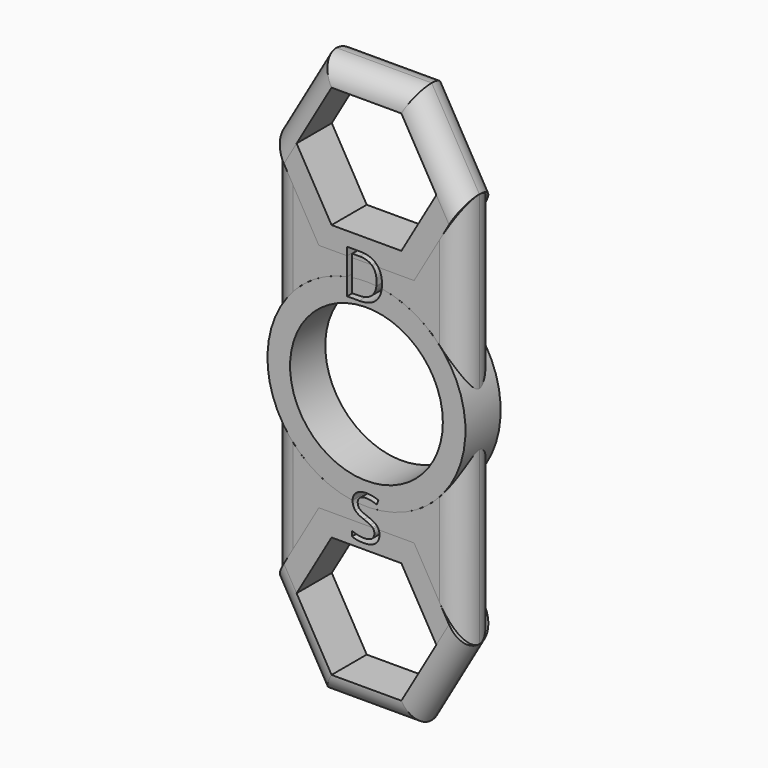
from build123d import *

# Parameters (mm, degrees)
F2_DEPTH = 6.35
F0_R     = 14.2875
F0_R_2   = 11.0236
F3_R     = 3.17499
F3_2_R   = 3.17499
F3_3_R   = 3.17499
F3_4_R   = 3.17499
F6_DEPTH = 25.4
F7_DEPTH = 25.4


# Not quite as in the source:
# - a fillet or chamfer is up to 0.001 mm smaller than in the source, because OpenCascade refuses the exact size


with BuildPart() as f2:
    # F1 (on Front) → F2 (new body)
    with BuildSketch(Plane.XZ):
        with BuildLine():
            Line((13.7481532851, -28.575), (13.7481532851, -3.8885649667))
            ThreePointArc((13.7481532851, -3.8885649667), (0, -14.2875), (-13.7481532851, -3.8885649667))
            Line((-13.7481532851, -3.8885649667), (-13.7481532851, -28.575))
            Line((-13.7481532851, -28.575), (-10.3111149312, -22.6218749436))
            Line((-10.3111149312, -22.6218749436), (-6.8740766425, -16.66875))
            Line((-6.8740766425, -16.66875), (0, -16.66875))
            Line((0, -16.66875), (6.8740766425, -16.66875))
            Line((6.8740766425, -16.66875), (10.3111148375, -22.6218747812))
            Line((10.3111148375, -22.6218747812), (13.7481532851, -28.575))
        make_face()
    extrude(amount=F2_DEPTH)

    # F3#3 (radius 3.175 in the source; OpenCascade refuses exactly that, so slightly less here)
    f3_3_edges = [f2.edges().sort_by_distance(p)[0] for p in [
        (13.748153, -6.35, -16.231782),
        (-13.748153, -6.35, -16.231782),
        (13.748153, 0, -16.231782),
        (-13.748153, 0, -16.231782),
    ]]
    fillet(f3_3_edges, radius=F3_3_R)


with BuildPart() as f2b:
    # F1 (on Front) → F2, piece 2 (new body)
    with BuildSketch(Plane.XZ):
        with BuildLine():
            Line((13.7481532851, 3.8885649667), (13.7481532851, 28.575))
            Line((13.7481532851, 28.575), (10.3111149612, 22.6218749955))
            Line((10.3111149612, 22.6218749955), (6.8740766425, 16.66875))
            Line((6.8740766425, 16.66875), (0, 16.66875))
            Line((0, 16.66875), (-6.8740766425, 16.66875))
            Line((-6.8740766425, 16.66875), (-10.3111150377, 22.6218751279))
            Line((-10.3111150377, 22.6218751279), (-13.7481532851, 28.575))
            Line((-13.7481532851, 28.575), (-13.7481532851, 3.8885649667))
            ThreePointArc((-13.7481532851, 3.8885649667), (0, 14.2875), (13.7481532851, 3.8885649667))
        make_face()
    extrude(amount=F2_DEPTH)

    # F3#2 (radius 3.175 in the source; OpenCascade refuses exactly that, so slightly less here)
    f3_2_edges = [f2b.edges().sort_by_distance(p)[0] for p in [
        (13.748153, -6.35, 16.231782),
        (-13.748153, -6.35, 16.231782),
        (13.748153, 0, 16.231782),
        (-13.748153, 0, 16.231782),
    ]]
    fillet(f3_2_edges, radius=F3_2_R)


with BuildPart() as f2c:
    # F0 (on Front) → F2, piece 3 (new body)
    with BuildSketch(Plane.XZ):
        Circle(F0_R)
        Circle(F0_R_2, mode=Mode.SUBTRACT)
    extrude(amount=F2_DEPTH)


with BuildPart() as f2d:
    # F0 (on Front) → F2, piece 4 (new body)
    with BuildSketch(Plane.XZ):
        Polygon((6.8740766425, -16.66875), (-6.8740766425, -16.66875), (-13.7481532851, -28.575), (-6.8740766425, -40.48125), (6.8740766425, -40.48125), (13.7481532851, -28.575), align=None)
        Polygon((-10.0819790757, -28.575), (-5.0409895379, -19.84375), (5.0409895379, -19.84375), (10.0819790757, -28.575), (5.0409895379, -37.30625), (-5.0409895379, -37.30625), align=None, mode=Mode.SUBTRACT)
    extrude(amount=F2_DEPTH)

    # F3#4 (radius 3.175 in the source; OpenCascade refuses exactly that, so slightly less here)
    f3_4_edges = [f2d.edges().sort_by_distance(p)[0] for p in [
        (10.311115, -6.35, -34.528125),
        (0, -6.35, -40.48125),
        (-10.311115, -6.35, -34.528125),
        (10.311115, 0, -34.528125),
        (0, 0, -40.48125),
        (-10.311115, 0, -34.528125),
    ]]
    fillet(f3_4_edges, radius=F3_4_R)


with BuildPart() as f2e:
    # F0 (on Front) → F2, piece 5 (new body)
    with BuildSketch(Plane.XZ):
        Polygon((-6.8740766425, 40.48125), (-13.7481532851, 28.575), (-6.8740766425, 16.66875), (6.8740766425, 16.66875), (13.7481532851, 28.575), (6.8740766425, 40.48125), align=None)
        Polygon((-10.0819790757, 28.575), (-5.0409895379, 37.30625), (5.0409895379, 37.30625), (10.0819790757, 28.575), (5.0409895379, 19.84375), (-5.0409895379, 19.84375), align=None, mode=Mode.SUBTRACT)
    extrude(amount=F2_DEPTH)

    # F3 (radius 3.175 in the source; OpenCascade refuses exactly that, so slightly less here)
    f3_edges = [f2e.edges().sort_by_distance(p)[0] for p in [
        (-10.311115, -6.35, 34.528125),
        (0, -6.35, 40.48125),
        (10.311115, -6.35, 34.528125),
        (0, 0, 40.48125),
        (10.311115, 0, 34.528125),
        (-10.311115, 0, 34.528125),
    ]]
    fillet(f3_edges, radius=F3_R)


with BuildPart() as f6_tool:
    # F4 (on face) → F6 (new body)
    with BuildSketch(Plane.XZ.offset(6.35)):
        with BuildLine():
            Line((0.7356463616, 16.66875), (1.7117723609, 16.66875))
            add(Edge.make_bspline(
                [(1.4261315737, 17.0095994575), (1.5843296653, 16.8514013659), (1.7117723609, 16.66875)],
                knots=[0, 0, 0, 0.1944106639, 0.1944106639, 0.1944106639], degree=2))
            add(Edge.make_bspline(
                [(-0.8565886954, 17.8233310113), (0.6124000198, 17.8233310113), (1.4261315737, 17.0095994575)],
                knots=[0, 0, 0, 1, 1, 1], degree=2))
            Line((-0.8565886954, 17.8233310113), (-2.7858421677, 17.8233310113))
            Line((-2.7858421677, 17.8233310113), (-2.7858421677, 16.66875))
            Line((-2.7858421677, 16.66875), (-2.0541038864, 16.66875))
            Line((-2.0541038864, 16.66875), (-2.0541038864, 17.1894334419))
            Line((-2.0541038864, 17.1894334419), (-0.9902584003, 17.1894334419))
            add(Edge.make_bspline(
                [(0.7356463616, 16.66875), (0.1235530561, 17.1894334419), (-0.9902584003, 17.1894334419)],
                knots=[0.0867132539, 0.0867132539, 0.0867132539, 1, 1, 1], degree=2))
        make_face()
        with BuildLine():
            ThreePointArc((-2.7858421677, 14.0132701275), (-2.4207903425, 14.0809243435), (-2.0541038864, 14.13907046))
            Line((-2.0541038864, 14.13907046), (-2.0541038864, 16.66875))
            Line((-2.0541038864, 16.66875), (-2.7858421677, 16.66875))
            Line((-2.7858421677, 16.66875), (-2.7858421677, 14.0132701275))
        make_face()
        with BuildLine():
            add(Edge.make_bspline(
                [(2.2030186501, 14.1166343396), (2.0632995934, 13.0044799084), (1.3937476761, 12.3518303603)],
                knots=[0.2086754636, 0.2086754636, 0.2086754636, 1, 1, 1], degree=2))
            ThreePointArc((2.2030186501, 14.1166343396), (1.8208483174, 14.1709974121), (1.4373488308, 14.2150161656))
            add(Edge.make_bspline(
                [(0.8060143862, 12.8038268881), (1.329389377, 13.31517027), (1.4373488308, 14.2150161656)],
                knots=[0, 0, 0, 0.7937244697, 0.7937244697, 0.7937244697], degree=2))
            add(Edge.make_bspline(
                [(-1.1625131746, 12.1595940322), (0.1466231101, 12.1595940322), (0.8060143862, 12.8038268881)],
                knots=[0, 0, 0, 1, 1, 1], degree=2))
            Line((-1.1625131746, 12.1595940322), (-2.0541038864, 12.1595940322))
            Line((-2.0541038864, 12.1595940322), (-2.0541038864, 14.13907046))
            ThreePointArc((-2.0541038864, 14.13907046), (-2.4207903425, 14.0809243435), (-2.7858421677, 14.0132701275))
            Line((-2.7858421677, 14.0132701275), (-2.7858421677, 11.5270745009))
            Line((-2.7858421677, 11.5270745009), (-1.0412458135, 11.5270745009))
            add(Edge.make_bspline(
                [(1.3937476761, 12.3518303603), (0.5476322247, 11.5270745009), (-1.0412458135, 11.5270745009)],
                knots=[0, 0, 0, 1, 1, 1], degree=2))
        make_face()
        with BuildLine():
            add(Edge.make_bspline(
                [(2.2398631275, 14.7351474176), (2.2398631275, 14.4099139371), (2.2030186501, 14.1166343396)],
                knots=[0, 0, 0, 0.2086754636, 0.2086754636, 0.2086754636], degree=2))
            add(Edge.make_bspline(
                [(1.7117723609, 16.66875), (2.2398631275, 15.9118882642), (2.2398631275, 14.7351474176)],
                knots=[0.1944106639, 0.1944106639, 0.1944106639, 1, 1, 1], degree=2))
            Line((1.7117723609, 16.66875), (0.7356463616, 16.66875))
            add(Edge.make_bspline(
                [(0.847355532, 16.5651821398), (0.7937623941, 16.6193130015), (0.7356463616, 16.66875)],
                knots=[0, 0, 0, 0.0867132539, 0.0867132539, 0.0867132539], degree=2))
            add(Edge.make_bspline(
                [(1.4654056622, 14.7089646919), (1.4654056622, 15.9409308377), (0.847355532, 16.5651821398)],
                knots=[0, 0, 0, 1, 1, 1], degree=2))
            add(Edge.make_bspline(
                [(1.4373488308, 14.2150161656), (1.4654056622, 14.448870855), (1.4654056622, 14.7089646919)],
                knots=[0.7937244697, 0.7937244697, 0.7937244697, 1, 1, 1], degree=2))
            ThreePointArc((1.4373488308, 14.2150161656), (1.8208483174, 14.1709974121), (2.2030186501, 14.1166343396))
        make_face()
    extrude(amount=-F6_DEPTH)


with BuildPart() as f2b_1:
    add(f2b.part)

    # F6: cut by f6_tool
    add(f6_tool.part, mode=Mode.SUBTRACT)


with BuildPart() as f2c_1:
    add(f2c.part)

    # F6: cut by f6_tool
    add(f6_tool.part, mode=Mode.SUBTRACT)


with BuildPart() as f2e_1:
    add(f2e.part)

    # F6: cut by f6_tool
    add(f6_tool.part, mode=Mode.SUBTRACT)


with BuildPart() as f7_tool:
    # F5 (on face) → F7 (new body)
    with BuildSketch(Plane.XZ.offset(6.35)):
        with BuildLine():
            ThreePointArc((-2.0011550915, -14.1466616044), (-1.6310895837, -14.1940904259), (-1.2599118366, -14.2318403031))
            add(Edge.make_bspline(
                [(-1.2611806878, -14.1660674247), (-1.2611806878, -14.1995701631), (-1.2599118366, -14.2318403031)],
                knots=[0, 0, 0, 0.1025818921, 0.1025818921, 0.1025818921], degree=2))
            add(Edge.make_bspline(
                [(-0.9338966167, -13.4729142129), (-1.2611806878, -13.7223391261), (-1.2611806878, -14.1660674247)],
                knots=[0, 0, 0, 1, 1, 1], degree=2))
            add(Edge.make_bspline(
                [(-0.0250804274, -13.2234892997), (-0.6066125455, -13.2234892997), (-0.9338966167, -13.4729142129)],
                knots=[0, 0, 0, 1, 1, 1], degree=2))
            add(Edge.make_bspline(
                [(1.4907615865, -13.5500843518), (0.7107919684, -13.2234892997), (-0.0250804274, -13.2234892997)],
                knots=[0, 0, 0, 1, 1, 1], degree=2))
            Line((1.4907615865, -13.5500843518), (1.7195159267, -12.913430706))
            add(Edge.make_bspline(
                [(-0.0071659309, -12.5689211574), (0.9312780795, -12.5689211574), (1.7195159267, -12.913430706)],
                knots=[0, 0, 0, 1, 1, 1], degree=2))
            add(Edge.make_bspline(
                [(-1.4547950542, -12.9995580932), (-0.9084029101, -12.5689211574), (-0.0071659309, -12.5689211574)],
                knots=[0, 0, 0, 1, 1, 1], degree=2))
            add(Edge.make_bspline(
                [(-2.0011550915, -14.1466616044), (-1.996998776, -13.4268939395), (-1.4547950542, -12.9995580932)],
                knots=[0.0076655975, 0.0076655975, 0.0076655975, 1, 1, 1], degree=2))
        make_face()
        with BuildLine():
            Line((0.8911016261, -16.66875), (1.7757291997, -16.66875))
            add(Edge.make_bspline(
                [(1.5059200066, -16.2289906018), (1.6829305163, -16.4217353791), (1.7757291997, -16.66875)],
                knots=[0, 0, 0, 0.475744782, 0.475744782, 0.475744782], degree=2))
            add(Edge.make_bspline(
                [(0.1430402323, -15.4710695949), (1.1338496941, -15.8238473727), (1.5059200066, -16.2289906018)],
                knots=[0, 0, 0, 1, 1, 1], degree=2))
            add(Edge.make_bspline(
                [(-0.7333920594, -15.0859079195), (-0.4467601149, -15.2602297511), (0.1430402323, -15.4710695949)],
                knots=[0, 0, 0, 1, 1, 1], degree=2))
            add(Edge.make_bspline(
                [(-1.1406023458, -14.7021242824), (-1.0200240038, -14.9115860879), (-0.7333920594, -15.0859079195)],
                knots=[0, 0, 0, 1, 1, 1], degree=2))
            add(Edge.make_bspline(
                [(-1.2599118366, -14.2318403031), (-1.2488115334, -14.5141494652), (-1.1406023458, -14.7021242824)],
                knots=[0.1025818921, 0.1025818921, 0.1025818921, 1, 1, 1], degree=2))
            ThreePointArc((-1.2599118366, -14.2318403031), (-1.6310895837, -14.1940904259), (-2.0011550915, -14.1466616044))
            add(Edge.make_bspline(
                [(-2.0011871983, -14.1577991956), (-2.0011871983, -14.1522216749), (-2.0011550915, -14.1466616044)],
                knots=[0, 0, 0, 0.0076655975, 0.0076655975, 0.0076655975], degree=2))
            add(Edge.make_bspline(
                [(-1.6242937521, -15.2815893432), (-2.0011871983, -14.8509524074), (-2.0011871983, -14.1577991956)],
                knots=[0, 0, 0, 1, 1, 1], degree=2))
            add(Edge.make_bspline(
                [(-0.369589976, -16.0264189872), (-1.2474003059, -15.7122262789), (-1.6242937521, -15.2815893432)],
                knots=[0, 0, 0, 1, 1, 1], degree=2))
            add(Edge.make_bspline(
                [(0.5667869771, -16.4267390827), (0.2587954406, -16.2496611747), (-0.369589976, -16.0264189872)],
                knots=[0, 0, 0, 1, 1, 1], degree=2))
            add(Edge.make_bspline(
                [(0.8911016261, -16.66875), (0.7657491045, -16.5411311783), (0.5667869771, -16.4267390827)],
                knots=[0.3540013155, 0.3540013155, 0.3540013155, 1, 1, 1], degree=2))
        make_face()
        with BuildLine():
            add(Edge.make_bspline(
                [(1.8779903191, -17.279055706), (1.8779903191, -18.1100127372), (1.275098609, -18.575789647)],
                knots=[0, 0, 0, 1, 1, 1], degree=2))
            add(Edge.make_bspline(
                [(1.7757291997, -16.66875), (1.8779903191, -16.9409520479), (1.8779903191, -17.279055706)],
                knots=[0.475744782, 0.475744782, 0.475744782, 1, 1, 1], degree=2))
            Line((1.7757291997, -16.66875), (0.8911016261, -16.66875))
            add(Edge.make_bspline(
                [(1.0063811611, -16.8125897772), (0.9597936508, -16.7386839361), (0.8911016261, -16.66875)],
                knots=[0, 0, 0, 0.3540013155, 0.3540013155, 0.3540013155], degree=2))
            add(Edge.make_bspline(
                [(1.1379838087, -17.3479576157), (1.1379838087, -17.0213625636), (1.0063811611, -16.8125897772)],
                knots=[0, 0, 0, 1, 1, 1], degree=2))
            add(Edge.make_bspline(
                [(0.7672915344, -18.1217260619), (1.1379838087, -17.8440513657), (1.1379838087, -17.3479576157)],
                knots=[0, 0, 0, 1, 1, 1], degree=2))
            add(Edge.make_bspline(
                [(-0.3351390212, -18.3994007581), (0.3965992601, -18.3994007581), (0.7672915344, -18.1217260619)],
                knots=[0, 0, 0, 1, 1, 1], degree=2))
            add(Edge.make_bspline(
                [(-1.2391320767, -18.3043161227), (-0.7830014344, -18.3994007581), (-0.3351390212, -18.3994007581)],
                knots=[0, 0, 0, 1, 1, 1], degree=2))
            add(Edge.make_bspline(
                [(-2.0838694899, -18.0466229803), (-1.6952627191, -18.2092314872), (-1.2391320767, -18.3043161227)],
                knots=[0, 0, 0, 1, 1, 1], degree=2))
            Line((-2.0838694899, -18.0466229803), (-2.0838694899, -18.7521785359))
            add(Edge.make_bspline(
                [(-0.3613217469, -19.0415665567), (-1.4802887608, -19.0415665567), (-2.0838694899, -18.7521785359)],
                knots=[0, 0, 0, 1, 1, 1], degree=2))
            add(Edge.make_bspline(
                [(1.275098609, -18.575789647), (0.672206899, -19.0415665567), (-0.3613217469, -19.0415665567)],
                knots=[0, 0, 0, 1, 1, 1], degree=2))
        make_face()
    extrude(amount=-F7_DEPTH)


with BuildPart() as f2_1:
    add(f2.part)

    # F7: cut by f7_tool
    add(f7_tool.part, mode=Mode.SUBTRACT)


with BuildPart() as f2c_2:
    add(f2c_1.part)

    # F7: cut by f7_tool
    add(f7_tool.part, mode=Mode.SUBTRACT)


with BuildPart() as f2d_1:
    add(f2d.part)

    # F7: cut by f7_tool
    add(f7_tool.part, mode=Mode.SUBTRACT)


solid = Compound([f2b_1.part, f2e_1.part, f2_1.part, f2c_2.part, f2d_1.part])
